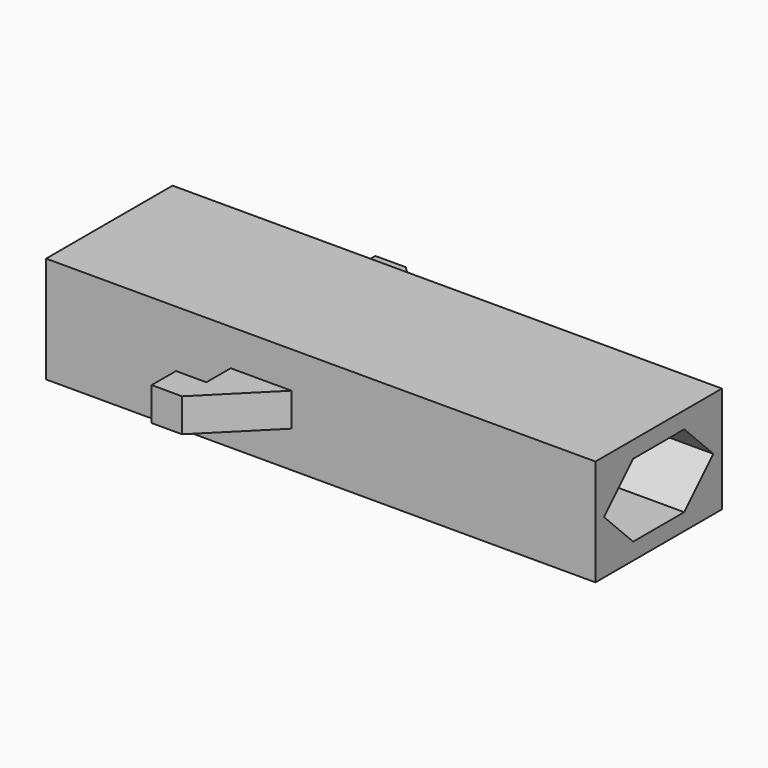
from build123d import *

# Parameters (mm, degrees)
F1_DEPTH  = 10
F2_W      = 21
F2_H      = 10
F3_DEPTH  = 9
F4_DEPTH  = 2
F5_DEPTH  = 3
F6_DEPTH  = 5
F7_DEPTH  = 2.5
F8_W      = 22.5
F8_H      = 12
F9_DEPTH  = 75
F11_DEPTH = 12
F12_SIZE  = 5.99999
F13_W     = 15
F13_H     = 5.5
F14_DEPTH = 10
F15_SIZE  = 9.99999
F16_W     = 5
F16_H     = 5.5
F17_DEPTH = 5
F18_W     = 15
F18_H     = 5.5
F19_DEPTH = 10
F20_SIZE  = 9.99999
F21_W     = 5
F21_H     = 5.5
F22_DEPTH = 5
F23_DEPTH = 5
F24_SIZE  = 5
F25_DEPTH = 5
F29_DEPTH = 25


# Not quite as in the source:
# - a fillet or chamfer is up to 0.001 mm smaller than in the source, because OpenCascade refuses the exact size
# - a feature of the source that left no trace in its solid (it failed there, or was rolled back) is left out


with BuildPart() as f1:
    # F0 (on Top) → F1 (new body)
    with BuildSketch(Plane.XY):
        Polygon((0, 10.5), (0, 0), (15, 0), align=None)
        Polygon((0, 10.5), (15, 0), (91, 0), (91, 21), (15, 21), align=None)
        Polygon((0, 21), (0, 10.5), (15, 21), align=None)
    extrude(amount=F1_DEPTH)

    # F2 (on face) → F3 (join)
    with BuildSketch(Plane(origin=(0, 0, 0), x_dir=(0, -1, 0), z_dir=(-1, 0, 0))):
        with Locations((-10.5, 5)):
            Rectangle(F2_W, F2_H)
    extrude(amount=F3_DEPTH)

    # F4 (add): a face of the model
    f4_faces = [f1.faces().sort_by_distance(p)[0] for p in [
        (41, 10.5, 10),
    ]]
    extrude(f4_faces, amount=F4_DEPTH)

    # F5 (add): a face of the model
    f5_faces = [f1.faces().sort_by_distance(p)[0] for p in [
        (41, 10.5, 12),
    ]]
    extrude(f5_faces, amount=F5_DEPTH)

    # F6 (add): a face of the model
    f6_faces = [f1.faces().sort_by_distance(p)[0] for p in [
        (41, 21, 7.5),
    ]]
    extrude(f6_faces, amount=F6_DEPTH)

    # F7 (add): a face of the model
    f7_faces = [f1.faces().sort_by_distance(p)[0] for p in [
        (41, 13, 15),
    ]]
    extrude(f7_faces, amount=F7_DEPTH)

    # F8 (on face) → F9 (cut)
    with BuildSketch(Plane.YZ.offset(91)):
        with Locations((13, 8.75)):
            Rectangle(F8_W, F8_H)
    extrude(amount=-F9_DEPTH, mode=Mode.SUBTRACT)

    # F10 (on face) → F11 (cut)
    with BuildSketch(Plane.XY.offset(2.75)):
        Polygon((16, 1.75), (16, 13), (1, 13), align=None)
        Polygon((1, 13), (16, 13), (16, 24.25), align=None)
    extrude(amount=F11_DEPTH, mode=Mode.SUBTRACT)

    # F12 (size 6 in the source; OpenCascade refuses exactly that, so slightly less here)
    f12_edges = [f1.edges().sort_by_distance(p)[0] for p in [
        (8.5, 7.375, 14.75),
        (8.5, 18.625, 14.75),
        (8.5, 7.375, 2.75),
        (8.5, 18.625, 2.75),
        (53.5, 1.75, 2.75),
        (53.5, 1.75, 14.75),
        (53.5, 24.25, 14.75),
        (53.5, 24.25, 2.75),
    ]]
    chamfer(f12_edges, length=F12_SIZE)

    # F13 (on face) → F14 (join)
    with BuildSketch(Plane(origin=(0, 26, 0), x_dir=(-1, 0, 0), z_dir=(0, 1, 0))):
        with Locations((-33.5, 8.75)):
            Rectangle(F13_W, F13_H)
    extrude(amount=F14_DEPTH)

    # F15 (size 10 in the source; OpenCascade refuses exactly that, so slightly less here)
    f15_edges = [f1.edges().sort_by_distance(p)[0] for p in [
        (41, 36, 8.75),
    ]]
    chamfer(f15_edges, length=F15_SIZE)

    # F16 (on face) → F17 (cut)
    with BuildSketch(Plane(origin=(26, 0, 0), x_dir=(0, -1, 0), z_dir=(-1, 0, 0))):
        with Locations((-28.5, 8.75)):
            Rectangle(F16_W, F16_H)
    extrude(amount=-F17_DEPTH, mode=Mode.SUBTRACT)

    # F18 (on face) → F19 (join)
    with BuildSketch(Plane.XZ):
        with Locations((33.5, 8.75)):
            Rectangle(F18_W, F18_H)
    extrude(amount=F19_DEPTH)

    # F20 (size 10 in the source; OpenCascade refuses exactly that, so slightly less here)
    f20_edges = [f1.edges().sort_by_distance(p)[0] for p in [
        (41, -10, 8.75),
    ]]
    chamfer(f20_edges, length=F20_SIZE)

    # F21 (on face) → F22 (cut)
    with BuildSketch(Plane(origin=(26, 0, 0), x_dir=(0, -1, 0), z_dir=(-1, 0, 0))):
        with Locations((2.5, 8.75)):
            Rectangle(F21_W, F21_H)
    extrude(amount=-F22_DEPTH, mode=Mode.SUBTRACT)

    # F23 (add): a face of the model
    f23_faces = [f1.faces().sort_by_distance(p)[0] for p in [
        (-9, 13, 8.75),
    ]]
    extrude(f23_faces, amount=F23_DEPTH)

    # F24
    f24_edges = [f1.edges().sort_by_distance(p)[0] for p in [
        (-14, 26, 8.75),
        (-14, 13, 17.5),
        (-14, 0, 8.75),
        (-14, 13, 0),
    ]]
    chamfer(f24_edges, length=F24_SIZE)

    # F25 (add): a face of the model
    f25_faces = [f1.faces().sort_by_distance(p)[0] for p in [
        (-14, 13, 8.75),
    ]]
    extrude(f25_faces, amount=F25_DEPTH)

    # F28 (on face) → F29 (cut)
    with BuildSketch(Plane.XY.offset(17.5)):
        Polygon((-36.3743491471, 0), (0.634705736, 0), (0.634705736, 13), (0.634705736, 34.4582907856), (-36.3743491471, 34.4582907856), align=None)
    extrude(amount=-F29_DEPTH, mode=Mode.SUBTRACT)


solid = f1.part
